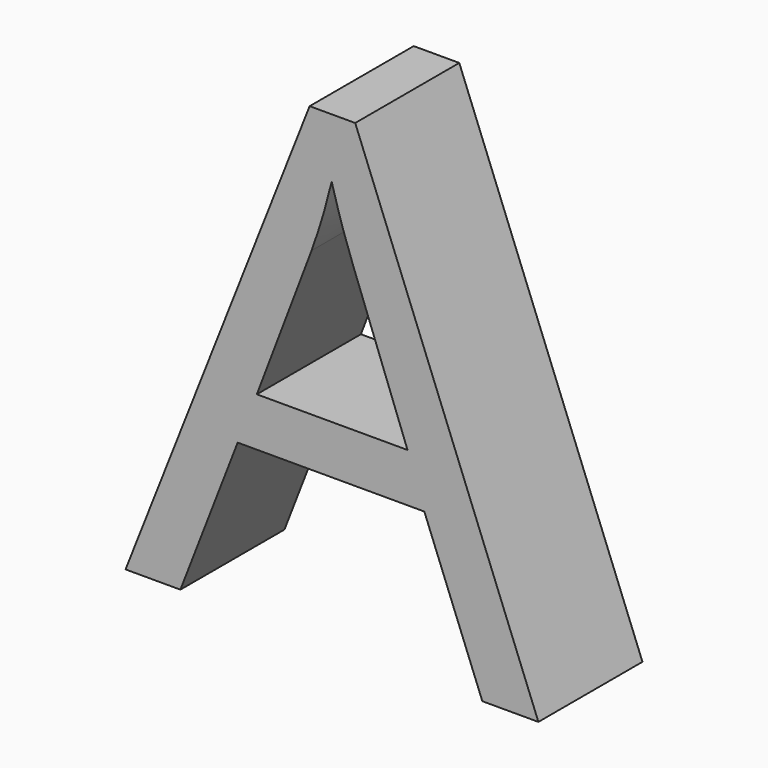
from build123d import *

# Parameters (mm, degrees)
F0_TEXT_SIZE = 125.3838340441
F1_DEPTH     = 25


# Not quite as in the source:
# - Text() gives the source's letters only with a copy of the font that has no kerning and outlines rounded to 1/6400 em; it was checked with that copy


with BuildPart() as f1:
    # F0 (on Front) → F1 (new body)
    with BuildSketch(Plane.XZ):
        with Locations((-48.9265620708, -42.4799285829)):
            Text('A', F0_TEXT_SIZE, font='Open Sans', text_align=(TextAlign.LEFT, TextAlign.BOTTOM))
    extrude(amount=F1_DEPTH)


solid = f1.part
